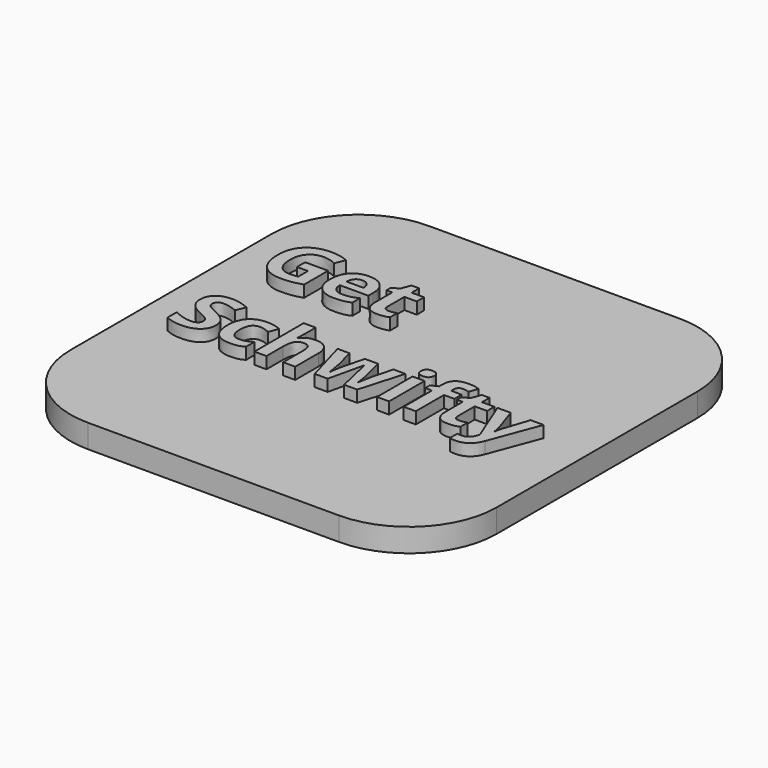
from build123d import *

# Parameters (mm, degrees)
F0_W         = 36.5
F0_H         = 36.5
F1_DEPTH     = 2
F2_TEXT_SIZE = 6.9444444444
F3_DEPTH     = 1
F4_R         = 7.5


# Not quite as in the source:
# - Text() gives the source's letters only with a copy of the font that has no kerning and outlines rounded to 1/6400 em; it was checked with that copy


with BuildPart() as f1:
    # F0 (on Top) → F1 (new body)
    with BuildSketch(Plane.XY):
        Rectangle(F0_W, F0_H)
    extrude(amount=F1_DEPTH)

    # F2 (on face) → F3 (join)
    with BuildSketch(Plane.XY.offset(2)):
        with Locations((-15.2404365543, 4.6938613258)):
            Text('Get', F2_TEXT_SIZE, font='Open Sans', font_style=FontStyle.BOLD, text_align=(TextAlign.LEFT, TextAlign.BOTTOM))
        with Locations((-15.2404365543, -4.7505831186)):
            Text('Schwifty', F2_TEXT_SIZE, font='Open Sans', font_style=FontStyle.BOLD, text_align=(TextAlign.LEFT, TextAlign.BOTTOM))
    extrude(amount=F3_DEPTH)

    # F4
    f4_edges = [f1.edges().sort_by_distance(p)[0] for p in [
        (18.25, 18.25, 1),
        (-18.25, 18.25, 1),
        (-18.25, -18.25, 1),
        (18.25, -18.25, 1),
    ]]
    fillet(f4_edges, radius=F4_R)


solid = f1.part
